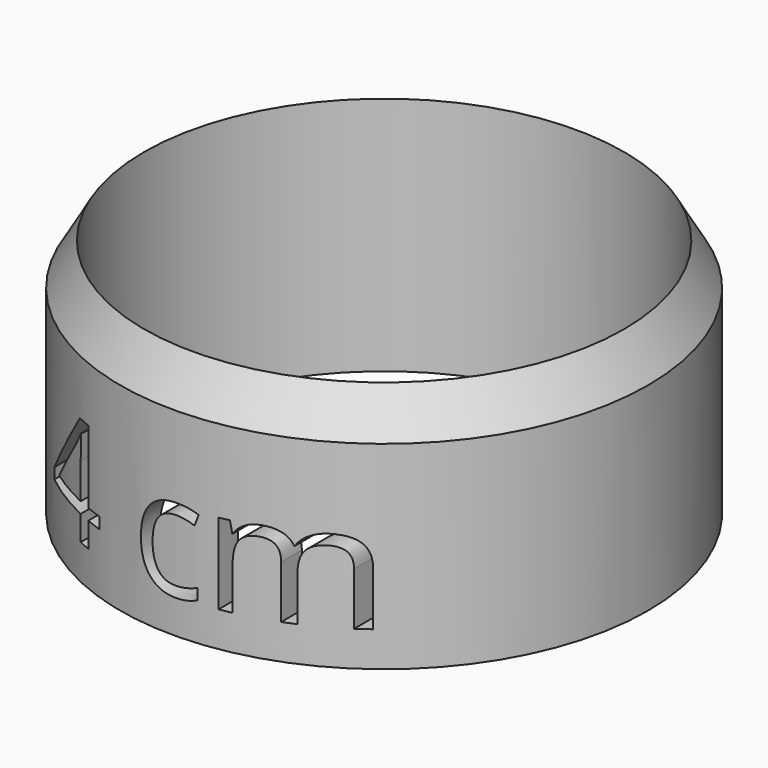
from build123d import *

# Parameters (mm, degrees)
F0_R         = 22
F0_R_2       = 20
F1_DEPTH     = 20
F2_TEXT_SIZE = 12.6037417358
F3_DEPTH     = 23.0000001002
F4_SIZE2     = 3.464092
F4_SIZE      = 1.99999


# Not quite as in the source:
# - a fillet or chamfer is up to 0.001 mm smaller than in the source, because OpenCascade refuses the exact size
# - Text() gives the source's letters only with a copy of the font that has no kerning and outlines rounded to 1/6400 em; it was checked with that copy


with BuildPart() as f1:
    # F0 (on Top) → F1 (new body)
    with BuildSketch(Plane.XY):
        Circle(F0_R)
        Circle(F0_R_2, mode=Mode.SUBTRACT)
    extrude(amount=F1_DEPTH)

    # F2 (on Front) → F3 (cut, up to face)
    with BuildSketch(Plane.XZ):
        with Locations((-14, 2.9253059502)):
            Text('4 cm', F2_TEXT_SIZE, font='Open Sans', text_align=(TextAlign.LEFT, TextAlign.BOTTOM))
    extrude(amount=F3_DEPTH, mode=Mode.SUBTRACT)

    # F4 (size 2 and 3.4641016151 in the source; OpenCascade refuses exactly that, so slightly less here)
    f4_edges = [f1.edges().sort_by_distance(p)[0] for p in [
        (-22, 0, 20),
    ]]
    f4_side = f1.faces().sort_by_distance((-21.377746, 0, 20))[0]
    chamfer(f4_edges, length=F4_SIZE, length2=F4_SIZE2, reference=f4_side)


solid = f1.part
